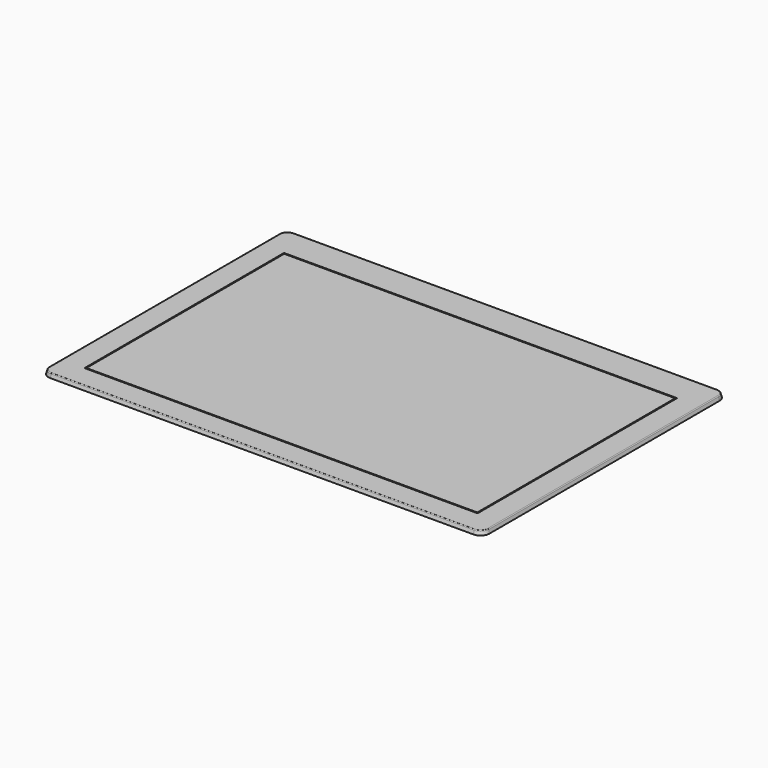
from build123d import *

# Parameters (mm, degrees)
F0_W                   = 219
F0_H                   = 138.5
F1_DEPTH               = 2.25
DRAFT_F1_DRAFTED_ANGLE = 15
F2_DEPTH               = 2.25
F3_R                   = 0.5


# Not quite as in the source:
# - an extrude with a draft is written as a straight extrude whose walls are then drafted


with BuildPart() as f1:
    # F0 (on Top) → F1 (new body)
    with BuildSketch(Plane.XY):
        with BuildLine():
            Line((-118.5, -85.5), (118.5, -85.5))
            ThreePointArc((118.5, -85.5), (122.0355339059, -84.0355339059), (123.5, -80.5))
            Line((123.5, -80.5), (123.5, 80.5))
            ThreePointArc((123.5, 80.5), (122.0355339059, 84.0355339059), (118.5, 85.5))
            Line((118.5, 85.5), (-118.5, 85.5))
            ThreePointArc((-118.5, 85.5), (-122.0355339059, 84.0355339059), (-123.5, 80.5))
            Line((-123.5, 80.5), (-123.5, -80.5))
            ThreePointArc((-123.5, -80.5), (-122.0355339059, -84.0355339059), (-118.5, -85.5))
        make_face()
        with Locations((0, -2.25)):
            Rectangle(F0_W, F0_H, mode=Mode.SUBTRACT)
    extrude(amount=F1_DEPTH)

    # draft_F1_drafted
    draft_f1_drafted_walls = [f1.faces().sort_by_distance(p)[0] for p in [
        (-123.5, 0, 1.5),
        (-122.0355339059, -84.0355339059, 1.5),
        (0, -85.5, 1.5),
        (122.0355339059, -84.0355339059, 1.5),
        (123.5, 0, 1.5),
        (122.0355339059, 84.0355339059, 1.5),
        (0, 85.5, 1.5),
        (-122.0355339059, 84.0355339059, 1.5),
        (-109.5, -2.25, 1.5),
        (0, 67, 1.5),
        (109.5, -2.25, 1.5),
        (0, -71.5, 1.5),
    ]]
    draft(draft_f1_drafted_walls, neutral_plane=Plane.XY, angle=DRAFT_F1_DRAFTED_ANGLE)

    # F3
    f3_edges = [f1.edges().sort_by_distance(p)[0] for p in [
        (-122.897114, 0, 2.25),
        (-121.609229, -83.609229, 2.25),
        (0, -84.897114, 2.25),
        (121.609229, -83.609229, 2.25),
        (122.897114, 0, 2.25),
        (121.609229, 83.609229, 2.25),
        (0, 84.897114, 2.25),
        (-121.609229, 83.609229, 2.25),
    ]]
    fillet(f3_edges, radius=F3_R)


with BuildPart() as f2:
    # F0 (on Top) → F2 (new body, through all)
    with BuildSketch(Plane.XY):
        with Locations((0, -2.25)):
            Rectangle(F0_W, F0_H)
    extrude(amount=F2_DEPTH)


solid = Compound([f1.part, f2.part])
